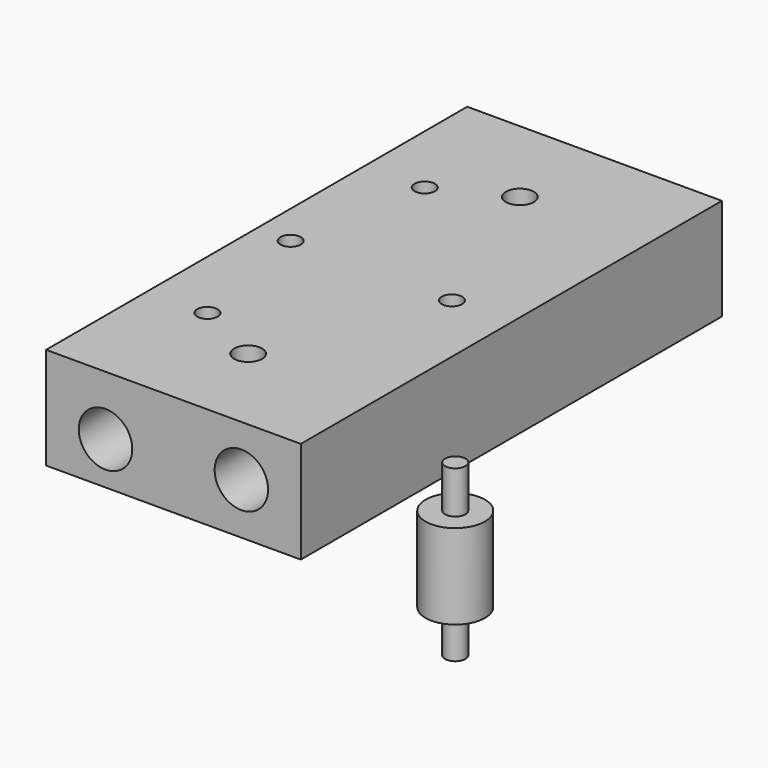
from build123d import *

# Parameters (mm, degrees)
F0_W      = 30
F0_H      = 12
F1_DEPTH  = 62
F2_D      = 6.3
F2_DEPTH  = 60
F2_TIP    = 1.8927109499
F3_D      = 6.3
F3_DEPTH  = 51
F3_TIP    = 1.8927109499
F5_D      = 3.3
F6_R      = 1.2
F7_DEPTH  = 10
F6_R_2    = 3.5
F8_DEPTH  = 5
F10_D     = 2
F10_DEPTH = 8
F10_TIP   = 0.600860619
F12_D     = 2.4
F12_DEPTH = 8
F12_TIP   = 0.7210327428
F13_D     = 2.4
F13_DEPTH = 3
F13_TIP   = 0.7210327428
F14_D     = 3


# Not quite as in the source:
# - a feature names something its author has since deleted; it is built from what else it names


with BuildPart() as f1:
    # F0 (on Front) → F1 (new body)
    with BuildSketch(Plane.XZ):
        Rectangle(F0_W, F0_H)
    extrude(amount=-F1_DEPTH)

    # F2
    with Locations(Plane.XZ):
        with Locations((-8, -1)):
            Hole(F2_D / 2, depth=F2_DEPTH)
            with Locations((0, 0, -(F2_DEPTH + F2_TIP / 2))):  # 118° drill point
                Cone(0, F2_D / 2, F2_TIP, mode=Mode.SUBTRACT)

    # F3
    with Locations(Plane.XZ):
        with Locations((8, 0)):
            Hole(F3_D / 2, depth=F3_DEPTH)
            with Locations((0, 0, -(F3_DEPTH + F3_TIP / 2))):  # 118° drill point
                Cone(0, F3_D / 2, F3_TIP, mode=Mode.SUBTRACT)

    # F5 (through all)
    with Locations(Plane(origin=(0, 0, -6), x_dir=(1, 0, 0), z_dir=(0, 0, -1))):
        with Locations((0, -11), (0, -51)):
            Hole(F5_D / 2)

    # F10
    with Locations(Plane(origin=(-15, 0, 0), x_dir=(0, -1, 0), z_dir=(-1, 0, 0))):
        with Locations((-31, 3.5)):
            Hole(F10_D / 2, depth=F10_DEPTH)
            with Locations((0, 0, -(F10_DEPTH + F10_TIP / 2))):  # 118° drill point
                Cone(0, F10_D / 2, F10_TIP, mode=Mode.SUBTRACT)

    # F12
    with Locations(Plane.XY.offset(6)):
        with Locations((-8, 15), (-8, 47), (8, 31)):
            Hole(F12_D / 2, depth=F12_DEPTH)
            with Locations((0, 0, -(F12_DEPTH + F12_TIP / 2))):  # 118° drill point
                Cone(0, F12_D / 2, F12_TIP, mode=Mode.SUBTRACT)

    # F13
    with Locations(Plane.XY.offset(6)):
        with Locations((-11, 31)):
            Hole(F13_D / 2, depth=F13_DEPTH)
            with Locations((0, 0, -(F13_DEPTH + F13_TIP / 2))):  # 118° drill point
                Cone(0, F13_D / 2, F13_TIP, mode=Mode.SUBTRACT)

    # F14 (through all)
    with Locations(Plane.XZ):
        with Locations((-8, -1), (8, 0)):
            Hole(F14_D / 2)


with BuildPart() as f7:
    # F6 (on Top) → F7 (new body, symmetric)
    with BuildSketch(Plane.XY):
        with Locations((33.1928394735, 0)):
            Circle(F6_R)
    extrude(amount=F7_DEPTH, both=True)

    # F6 (on Top) → F8 (join, symmetric)
    with BuildSketch(Plane.XY):
        with Locations((33.1928394735, 0)):
            Circle(F6_R_2)
        with Locations((33.1928394735, 0)):
            Circle(F6_R, mode=Mode.SUBTRACT)
    extrude(amount=F8_DEPTH, both=True)


solid = Compound([f1.part, f7.part])
